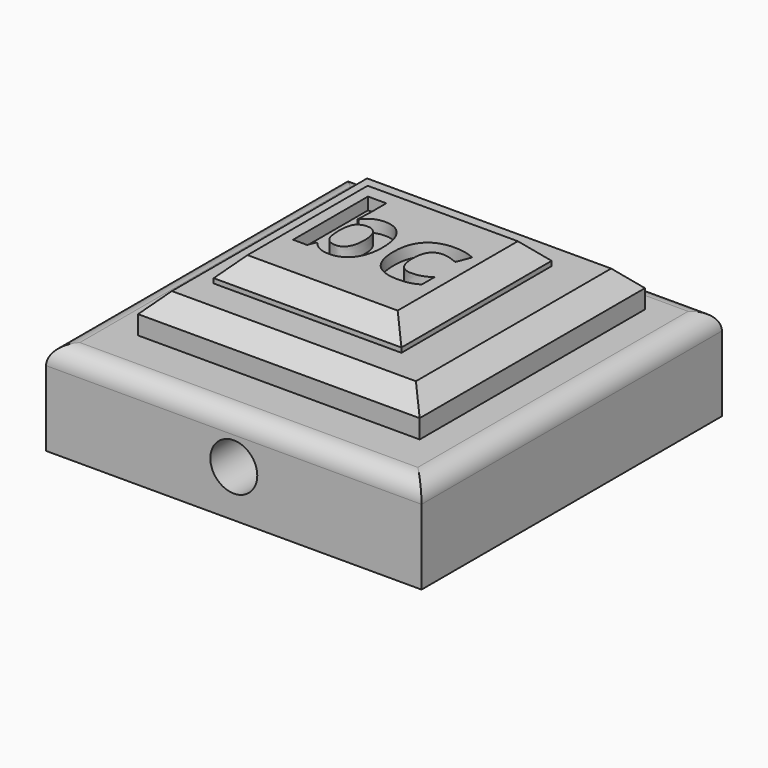
from build123d import *

# Parameters (mm, degrees)
F0_W         = 101.6
F0_H         = 101.6
F1_DEPTH     = 25.4
F2_W         = 76.2
F2_H         = 76.2
F3_DEPTH     = 10.16
F4_W         = 50.8
F4_H         = 50.8
F5_DEPTH     = 6.35
F6_TEXT_SIZE = 33.3467443092
F7_DEPTH     = 3.302
F8_R         = 6.35
F9_DEPTH     = 122.682
F10_R        = 5.08
F11_SIZE     = 5.08
F12_SIZE     = 5.08


# Not quite as in the source:
# - Text() gives the source's letters only with a copy of the font that has no kerning and outlines rounded to 1/6400 em; it was checked with that copy


with BuildPart() as f1:
    # F0 (on Top) → F1 (new body)
    with BuildSketch(Plane.XY):
        with Locations((0, 50.8)):
            Rectangle(F0_W, F0_H)
    extrude(amount=F1_DEPTH)

    # F2 (on face) → F3 (join)
    with BuildSketch(Plane.XY.offset(25.4)):
        with Locations((-0.0478215516, 53.39943182)):
            Rectangle(F2_W, F2_H)
    extrude(amount=F3_DEPTH)

    # F4 (on face) → F5 (join)
    with BuildSketch(Plane.XY.offset(35.56)):
        with Locations((-2.933989279, 54.0142105608)):
            Rectangle(F4_W, F4_H)
    extrude(amount=F5_DEPTH)

    # F6 (on face) → F7 (cut)
    with BuildSketch(Plane.XY.offset(41.91)):
        with Locations((-22.728510816, 45.192915105)):
            Text('bc', F6_TEXT_SIZE, font='Open Sans', font_style=FontStyle.BOLD, text_align=(TextAlign.LEFT, TextAlign.BOTTOM))
    extrude(amount=-F7_DEPTH, mode=Mode.SUBTRACT)

    # F8 (on face) → F9 (cut)
    with BuildSketch(Plane.XZ):
        with Locations((0, 12.710949406)):
            Circle(F8_R)
    extrude(amount=-F9_DEPTH, mode=Mode.SUBTRACT)

    # F10
    f10_edges = [f1.edges().sort_by_distance(p)[0] for p in [
        (-50.8, 50.8, 25.4),
        (0, 101.6, 25.4),
        (50.8, 50.8, 25.4),
        (0, 0, 25.4),
    ]]
    fillet(f10_edges, radius=F10_R)

    # F11
    f11_edges = [f1.edges().sort_by_distance(p)[0] for p in [
        (-0.047822, 91.499432, 35.56),
        (38.052178, 53.399432, 35.56),
        (-0.047822, 15.299432, 35.56),
        (-38.147822, 53.399432, 35.56),
    ]]
    chamfer(f11_edges, length=F11_SIZE)

    # F12
    f12_edges = [f1.edges().sort_by_distance(p)[0] for p in [
        (-2.933989, 79.414211, 41.91),
        (-28.333989, 54.014211, 41.91),
        (-2.933989, 28.614211, 41.91),
        (22.466011, 54.014211, 41.91),
    ]]
    chamfer(f12_edges, length=F12_SIZE)


solid = f1.part
